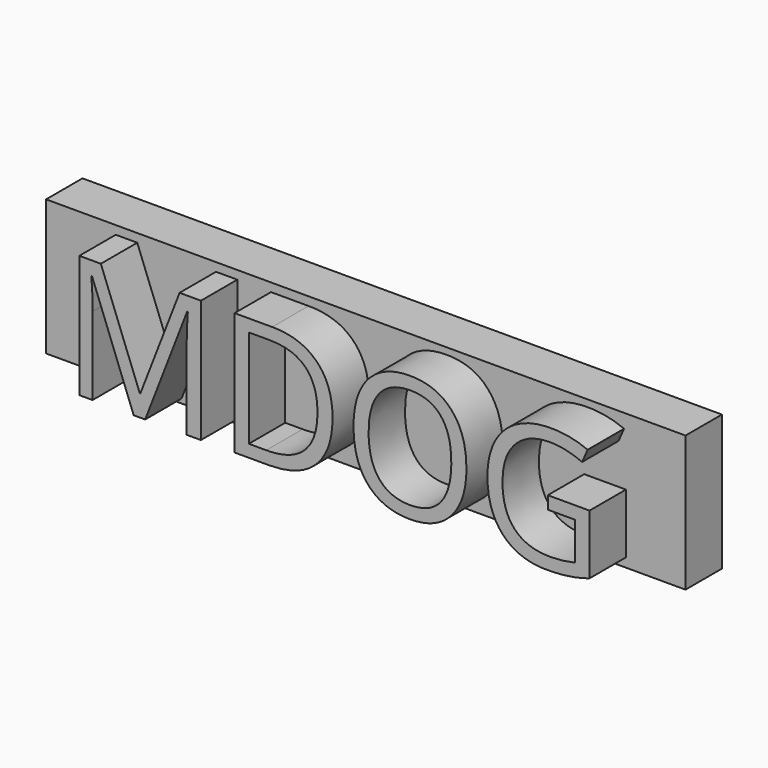
from build123d import *

# Parameters (mm, degrees)
F0_TEXT_SIZE = 23.9838121666
F1_DEPTH     = 6.35
F2_W         = 89.2054513097
F2_H         = 18.9305925742
F3_DEPTH     = 6.35


# Not quite as in the source:
# - Text() gives the source's letters only with a copy of the font that has no kerning and outlines rounded to 1/6400 em; it was checked with that copy


with BuildPart() as f1:
    # F0 (on Front) → F1 (new body)
    with BuildSketch(Plane.XZ):
        with Locations((-38.7098751962, 9.9292993546)):
            Text('MDOG', F0_TEXT_SIZE, font='Open Sans', text_align=(TextAlign.LEFT, TextAlign.BOTTOM))
    extrude(amount=F1_DEPTH)


with BuildPart() as f3:
    # F2 (on Front) → F3 (new body)
    with BuildSketch(Plane.XZ):
        with Locations((-1.4765001833, 18.7756917439)):
            Rectangle(F2_W, F2_H)
    extrude(amount=-F3_DEPTH)


solid = Compound([f1.part, f3.part])
